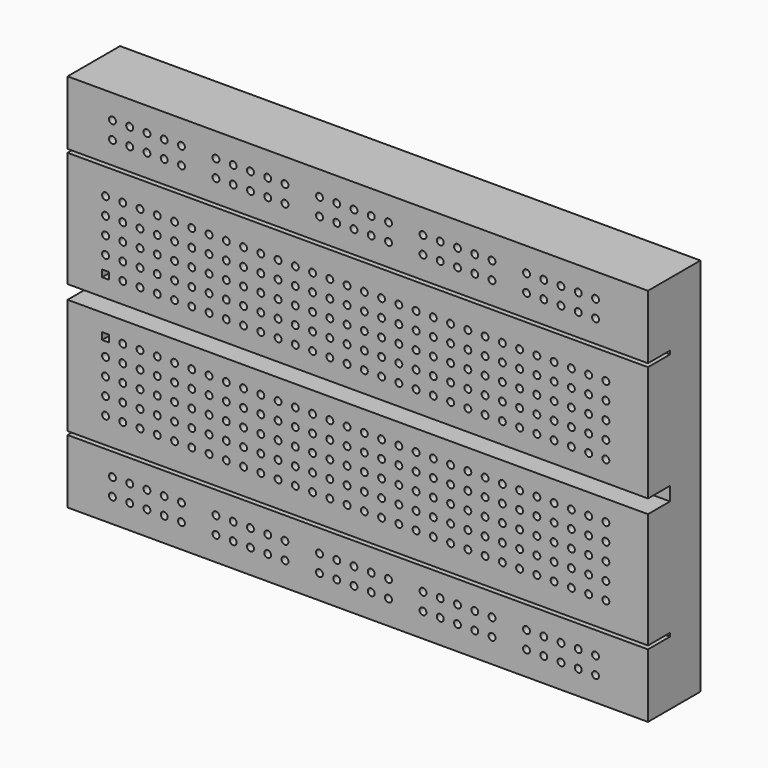
from build123d import *

# Parameters (mm, degrees)
F0_W     = 84.1
F0_H     = 55
F1_DEPTH = 9.5
F3_DEPTH = 5
F5_W     = 84.1
F5_H     = 2
F5_R     = 0.5
F5_H_2   = 0.5
F6_DEPTH = 4


with BuildPart() as f1:
    # F0 (on Front) → F1 (new body)
    with BuildSketch(Plane.XZ):
        Rectangle(F0_W, F0_H)
    extrude(amount=F1_DEPTH)

    # F2 (on face) → F3 (join)
    with BuildSketch(Plane(origin=(0, 0, 0), x_dir=(-1, 0, 0), z_dir=(0, 1, 0))):
        Polygon((44.05, 0), (42.05, 0), (42.05, -0.75), (44.05, -1.5), align=None)
        Polygon((44.05, 1.5), (42.05, 0.75), (42.05, 0), (44.05, 0), align=None)
        Polygon((1.5, -29.5), (0.75, -27.5), (-0.75, -27.5), (-1.5, -29.5), align=None)
    extrude(amount=-F3_DEPTH)

    # F5 (on face) → F6 (cut)
    with BuildSketch(Plane.XZ.offset(9.5)):
        Rectangle(F5_W, F5_H)
        with BuildLine():
            Line((-36.05, -4), (-36.05, -3.5))
            Line((-36.05, -3.5), (-36.55, -3.5))
            ThreePointArc((-36.55, -3.5), (-36.1964466094, -3.6464466094), (-36.05, -4))
        make_face()
        with BuildLine():
            ThreePointArc((-37.05, -4), (-36.9035533906, -3.6464466094), (-36.55, -3.5))
            Line((-36.55, -3.5), (-37.05, -3.5))
            Line((-37.05, -3.5), (-37.05, -4))
        make_face()
        with BuildLine():
            ThreePointArc((-36.05, -4), (-36.1964466094, -3.6464466094), (-36.55, -3.5))
            ThreePointArc((-36.55, -3.5), (-36.9035533906, -3.6464466094), (-37.05, -4))
            ThreePointArc((-37.05, -4), (-36.9035533906, -4.3535533906), (-36.55, -4.5))
            ThreePointArc((-36.55, -4.5), (-36.1964466094, -4.3535533906), (-36.05, -4))
        make_face()
        with BuildLine():
            Line((-36.05, -4.5), (-36.05, -4))
            ThreePointArc((-36.05, -4), (-36.1964466094, -4.3535533906), (-36.55, -4.5))
            Line((-36.55, -4.5), (-36.05, -4.5))
        make_face()
        with BuildLine():
            ThreePointArc((-36.55, -4.5), (-36.9035533906, -4.3535533906), (-37.05, -4))
            Line((-37.05, -4), (-37.05, -4.5))
            Line((-37.05, -4.5), (-36.55, -4.5))
        make_face()
        with Locations((-34.05, -4)):
            Circle(F5_R)
        with Locations((-31.55, -4)):
            Circle(F5_R)
        with Locations((-29.05, -4)):
            Circle(F5_R)
        with Locations((-26.55, -4)):
            Circle(F5_R)
        with Locations((-24.05, -4)):
            Circle(F5_R)
        with Locations((-21.55, -4)):
            Circle(F5_R)
        with Locations((-19.05, -4)):
            Circle(F5_R)
        with Locations((-16.55, -4)):
            Circle(F5_R)
        with Locations((-14.05, -4)):
            Circle(F5_R)
        with Locations((-11.55, -4)):
            Circle(F5_R)
        with Locations((-9.05, -4)):
            Circle(F5_R)
        with Locations((-6.55, -4)):
            Circle(F5_R)
        with Locations((-4.05, -4)):
            Circle(F5_R)
        with Locations((-1.55, -4)):
            Circle(F5_R)
        with Locations((0.95, -4)):
            Circle(F5_R)
        with Locations((3.45, -4)):
            Circle(F5_R)
        with Locations((5.95, -4)):
            Circle(F5_R)
        with Locations((8.45, -4)):
            Circle(F5_R)
        with Locations((10.95, -4)):
            Circle(F5_R)
        with Locations((13.45, -4)):
            Circle(F5_R)
        with Locations((15.95, -4)):
            Circle(F5_R)
        with Locations((18.45, -4)):
            Circle(F5_R)
        with Locations((20.95, -4)):
            Circle(F5_R)
        with Locations((23.45, -4)):
            Circle(F5_R)
        with Locations((25.95, -4)):
            Circle(F5_R)
        with Locations((28.45, -4)):
            Circle(F5_R)
        with Locations((30.95, -4)):
            Circle(F5_R)
        with Locations((33.45, -4)):
            Circle(F5_R)
        with Locations((35.95, -4)):
            Circle(F5_R)
        with Locations((25.95, -6.5)):
            Circle(F5_R)
        with Locations((28.45, -6.5)):
            Circle(F5_R)
        with Locations((-16.55, -6.5)):
            Circle(F5_R)
        with Locations((5.95, -6.5)):
            Circle(F5_R)
        with Locations((-31.55, -6.5)):
            Circle(F5_R)
        with Locations((20.95, -6.5)):
            Circle(F5_R)
        with Locations((-9.05, -6.5)):
            Circle(F5_R)
        with Locations((10.95, -6.5)):
            Circle(F5_R)
        with Locations((0.95, -6.5)):
            Circle(F5_R)
        with Locations((8.45, -6.5)):
            Circle(F5_R)
        with Locations((-14.05, -6.5)):
            Circle(F5_R)
        with Locations((-4.05, -6.5)):
            Circle(F5_R)
        with Locations((-11.55, -6.5)):
            Circle(F5_R)
        with Locations((15.95, -6.5)):
            Circle(F5_R)
        with Locations((3.45, -6.5)):
            Circle(F5_R)
        with Locations((13.45, -6.5)):
            Circle(F5_R)
        with Locations((-6.55, -6.5)):
            Circle(F5_R)
        with Locations((-29.05, -6.5)):
            Circle(F5_R)
        with Locations((18.45, -6.5)):
            Circle(F5_R)
        with Locations((23.45, -6.5)):
            Circle(F5_R)
        with Locations((30.95, -6.5)):
            Circle(F5_R)
        with Locations((33.45, -6.5)):
            Circle(F5_R)
        with Locations((-21.55, -6.5)):
            Circle(F5_R)
        with Locations((-26.55, -6.5)):
            Circle(F5_R)
        with Locations((-24.05, -6.5)):
            Circle(F5_R)
        with Locations((-19.05, -6.5)):
            Circle(F5_R)
        with Locations((35.95, -6.5)):
            Circle(F5_R)
        with Locations((-1.55, -6.5)):
            Circle(F5_R)
        with Locations((-34.05, -6.5)):
            Circle(F5_R)
        with Locations((-36.55, -6.5)):
            Circle(F5_R)
        with Locations((25.95, -9)):
            Circle(F5_R)
        with Locations((28.45, -9)):
            Circle(F5_R)
        with Locations((-16.55, -9)):
            Circle(F5_R)
        with Locations((5.95, -9)):
            Circle(F5_R)
        with Locations((-31.55, -9)):
            Circle(F5_R)
        with Locations((20.95, -9)):
            Circle(F5_R)
        with Locations((-9.05, -9)):
            Circle(F5_R)
        with Locations((10.95, -9)):
            Circle(F5_R)
        with Locations((0.95, -9)):
            Circle(F5_R)
        with Locations((8.45, -9)):
            Circle(F5_R)
        with Locations((-14.05, -9)):
            Circle(F5_R)
        with Locations((-4.05, -9)):
            Circle(F5_R)
        with Locations((-11.55, -9)):
            Circle(F5_R)
        with Locations((15.95, -9)):
            Circle(F5_R)
        with Locations((3.45, -9)):
            Circle(F5_R)
        with Locations((13.45, -9)):
            Circle(F5_R)
        with Locations((-6.55, -9)):
            Circle(F5_R)
        with Locations((-29.05, -9)):
            Circle(F5_R)
        with Locations((18.45, -9)):
            Circle(F5_R)
        with Locations((23.45, -9)):
            Circle(F5_R)
        with Locations((30.95, -9)):
            Circle(F5_R)
        with Locations((33.45, -9)):
            Circle(F5_R)
        with Locations((-21.55, -9)):
            Circle(F5_R)
        with Locations((-26.55, -9)):
            Circle(F5_R)
        with Locations((-24.05, -9)):
            Circle(F5_R)
        with Locations((-19.05, -9)):
            Circle(F5_R)
        with Locations((35.95, -9)):
            Circle(F5_R)
        with Locations((-1.55, -9)):
            Circle(F5_R)
        with Locations((-34.05, -9)):
            Circle(F5_R)
        with Locations((-36.55, -9)):
            Circle(F5_R)
        with Locations((25.95, -11.5)):
            Circle(F5_R)
        with Locations((28.45, -11.5)):
            Circle(F5_R)
        with Locations((-16.55, -11.5)):
            Circle(F5_R)
        with Locations((5.95, -11.5)):
            Circle(F5_R)
        with Locations((-31.55, -11.5)):
            Circle(F5_R)
        with Locations((20.95, -11.5)):
            Circle(F5_R)
        with Locations((-9.05, -11.5)):
            Circle(F5_R)
        with Locations((10.95, -11.5)):
            Circle(F5_R)
        with Locations((0.95, -11.5)):
            Circle(F5_R)
        with Locations((8.45, -11.5)):
            Circle(F5_R)
        with Locations((-14.05, -11.5)):
            Circle(F5_R)
        with Locations((-4.05, -11.5)):
            Circle(F5_R)
        with Locations((-11.55, -11.5)):
            Circle(F5_R)
        with Locations((15.95, -11.5)):
            Circle(F5_R)
        with Locations((3.45, -11.5)):
            Circle(F5_R)
        with Locations((13.45, -11.5)):
            Circle(F5_R)
        with Locations((-6.55, -11.5)):
            Circle(F5_R)
        with Locations((-29.05, -11.5)):
            Circle(F5_R)
        with Locations((18.45, -11.5)):
            Circle(F5_R)
        with Locations((23.45, -11.5)):
            Circle(F5_R)
        with Locations((30.95, -11.5)):
            Circle(F5_R)
        with Locations((33.45, -11.5)):
            Circle(F5_R)
        with Locations((-21.55, -11.5)):
            Circle(F5_R)
        with Locations((-26.55, -11.5)):
            Circle(F5_R)
        with Locations((-24.05, -11.5)):
            Circle(F5_R)
        with Locations((-19.05, -11.5)):
            Circle(F5_R)
        with Locations((35.95, -11.5)):
            Circle(F5_R)
        with Locations((-1.55, -11.5)):
            Circle(F5_R)
        with Locations((-34.05, -11.5)):
            Circle(F5_R)
        with Locations((-36.55, -11.5)):
            Circle(F5_R)
        with Locations((25.95, -14)):
            Circle(F5_R)
        with Locations((28.45, -14)):
            Circle(F5_R)
        with Locations((-16.55, -14)):
            Circle(F5_R)
        with Locations((5.95, -14)):
            Circle(F5_R)
        with Locations((-31.55, -14)):
            Circle(F5_R)
        with Locations((20.95, -14)):
            Circle(F5_R)
        with Locations((-9.05, -14)):
            Circle(F5_R)
        with Locations((10.95, -14)):
            Circle(F5_R)
        with Locations((0.95, -14)):
            Circle(F5_R)
        with Locations((8.45, -14)):
            Circle(F5_R)
        with Locations((-14.05, -14)):
            Circle(F5_R)
        with Locations((-4.05, -14)):
            Circle(F5_R)
        with Locations((-11.55, -14)):
            Circle(F5_R)
        with Locations((15.95, -14)):
            Circle(F5_R)
        with Locations((3.45, -14)):
            Circle(F5_R)
        with Locations((13.45, -14)):
            Circle(F5_R)
        with Locations((-6.55, -14)):
            Circle(F5_R)
        with Locations((-29.05, -14)):
            Circle(F5_R)
        with Locations((18.45, -14)):
            Circle(F5_R)
        with Locations((23.45, -14)):
            Circle(F5_R)
        with Locations((30.95, -14)):
            Circle(F5_R)
        with Locations((33.45, -14)):
            Circle(F5_R)
        with Locations((-21.55, -14)):
            Circle(F5_R)
        with Locations((-26.55, -14)):
            Circle(F5_R)
        with Locations((-24.05, -14)):
            Circle(F5_R)
        with Locations((-19.05, -14)):
            Circle(F5_R)
        with Locations((35.95, -14)):
            Circle(F5_R)
        with Locations((-1.55, -14)):
            Circle(F5_R)
        with Locations((-34.05, -14)):
            Circle(F5_R)
        with Locations((-36.55, -14)):
            Circle(F5_R)
        with Locations((0, -18)):
            Rectangle(F5_W, F5_H_2)
        with Locations((-35.55, -21.5)):
            Circle(F5_R)
        with Locations((-35.55, -24)):
            Circle(F5_R)
        with Locations((-33.05, -21.5)):
            Circle(F5_R)
        with Locations((-33.05, -24)):
            Circle(F5_R)
        with Locations((-30.55, -21.5)):
            Circle(F5_R)
        with Locations((-30.55, -24)):
            Circle(F5_R)
        with Locations((-28.05, -21.5)):
            Circle(F5_R)
        with Locations((-28.05, -24)):
            Circle(F5_R)
        with Locations((-25.55, -21.5)):
            Circle(F5_R)
        with Locations((-25.55, -24)):
            Circle(F5_R)
        with Locations((-18.05, -24)):
            Circle(F5_R)
        with Locations((-10.55, -24)):
            Circle(F5_R)
        with Locations((-13.05, -21.5)):
            Circle(F5_R)
        with Locations((-18.05, -21.5)):
            Circle(F5_R)
        with Locations((-15.55, -21.5)):
            Circle(F5_R)
        with Locations((-20.55, -24)):
            Circle(F5_R)
        with Locations((-13.05, -24)):
            Circle(F5_R)
        with Locations((-10.55, -21.5)):
            Circle(F5_R)
        with Locations((-15.55, -24)):
            Circle(F5_R)
        with Locations((-20.55, -21.5)):
            Circle(F5_R)
        with Locations((-3.05, -24)):
            Circle(F5_R)
        with Locations((4.45, -24)):
            Circle(F5_R)
        with Locations((1.95, -21.5)):
            Circle(F5_R)
        with Locations((-3.05, -21.5)):
            Circle(F5_R)
        with Locations((-0.55, -21.5)):
            Circle(F5_R)
        with Locations((-5.55, -24)):
            Circle(F5_R)
        with Locations((1.95, -24)):
            Circle(F5_R)
        with Locations((4.45, -21.5)):
            Circle(F5_R)
        with Locations((-0.55, -24)):
            Circle(F5_R)
        with Locations((-5.55, -21.5)):
            Circle(F5_R)
        with Locations((11.95, -24)):
            Circle(F5_R)
        with Locations((19.45, -24)):
            Circle(F5_R)
        with Locations((16.95, -21.5)):
            Circle(F5_R)
        with Locations((11.95, -21.5)):
            Circle(F5_R)
        with Locations((14.45, -21.5)):
            Circle(F5_R)
        with Locations((9.45, -24)):
            Circle(F5_R)
        with Locations((16.95, -24)):
            Circle(F5_R)
        with Locations((19.45, -21.5)):
            Circle(F5_R)
        with Locations((14.45, -24)):
            Circle(F5_R)
        with Locations((9.45, -21.5)):
            Circle(F5_R)
        with Locations((26.95, -24)):
            Circle(F5_R)
        with Locations((34.45, -24)):
            Circle(F5_R)
        with Locations((31.95, -21.5)):
            Circle(F5_R)
        with Locations((26.95, -21.5)):
            Circle(F5_R)
        with Locations((29.45, -21.5)):
            Circle(F5_R)
        with Locations((24.45, -24)):
            Circle(F5_R)
        with Locations((31.95, -24)):
            Circle(F5_R)
        with Locations((34.45, -21.5)):
            Circle(F5_R)
        with Locations((29.45, -24)):
            Circle(F5_R)
        with Locations((24.45, -21.5)):
            Circle(F5_R)
        with BuildLine():
            Line((-36.55, 3.5), (-36.05, 3.5))
            Line((-36.05, 3.5), (-36.05, 4))
            ThreePointArc((-36.05, 4), (-36.1964466094, 3.6464466094), (-36.55, 3.5))
        make_face()
        with BuildLine():
            Line((-37.05, 3.5), (-36.55, 3.5))
            ThreePointArc((-36.55, 3.5), (-36.9035533906, 3.6464466094), (-37.05, 4))
            Line((-37.05, 4), (-37.05, 3.5))
        make_face()
        with BuildLine():
            ThreePointArc((-37.05, 4), (-36.9035533906, 3.6464466094), (-36.55, 3.5))
            ThreePointArc((-36.55, 3.5), (-36.1964466094, 3.6464466094), (-36.05, 4))
            ThreePointArc((-36.05, 4), (-36.1964466094, 4.3535533906), (-36.55, 4.5))
            ThreePointArc((-36.55, 4.5), (-36.9035533906, 4.3535533906), (-37.05, 4))
        make_face()
        with BuildLine():
            ThreePointArc((-36.55, 4.5), (-36.1964466094, 4.3535533906), (-36.05, 4))
            Line((-36.05, 4), (-36.05, 4.5))
            Line((-36.05, 4.5), (-36.55, 4.5))
        make_face()
        with BuildLine():
            Line((-37.05, 4.5), (-37.05, 4))
            ThreePointArc((-37.05, 4), (-36.9035533906, 4.3535533906), (-36.55, 4.5))
            Line((-36.55, 4.5), (-37.05, 4.5))
        make_face()
        with Locations((-35.55, 21.5)):
            Circle(F5_R)
        with Locations((24.45, 21.5)):
            Circle(F5_R)
        with Locations((-20.55, 21.5)):
            Circle(F5_R)
        with Locations((-36.55, 6.5)):
            Circle(F5_R)
        with Locations((-5.55, 21.5)):
            Circle(F5_R)
        with Locations((9.45, 21.5)):
            Circle(F5_R)
        with Locations((-20.55, 24)):
            Circle(F5_R)
        with Locations((-35.55, 24)):
            Circle(F5_R)
        with Locations((-36.55, 11.5)):
            Circle(F5_R)
        with Locations((-3.05, 21.5)):
            Circle(F5_R)
        with Locations((-5.55, 24)):
            Circle(F5_R)
        with Locations((-36.55, 9)):
            Circle(F5_R)
        with Locations((26.95, 21.5)):
            Circle(F5_R)
        with Locations((-11.55, 4)):
            Circle(F5_R)
        with Locations((0, 18)):
            Rectangle(F5_W, F5_H_2)
        with Locations((11.95, 21.5)):
            Circle(F5_R)
        with Locations((-18.05, 21.5)):
            Circle(F5_R)
        with Locations((-34.05, 4)):
            Circle(F5_R)
        with Locations((-36.55, 14)):
            Circle(F5_R)
        with Locations((9.45, 24)):
            Circle(F5_R)
        with Locations((24.45, 24)):
            Circle(F5_R)
        with Locations((-33.05, 21.5)):
            Circle(F5_R)
        with Locations((-18.05, 24)):
            Circle(F5_R)
        with Locations((3.45, 4)):
            Circle(F5_R)
        with Locations((-26.55, 9)):
            Circle(F5_R)
        with Locations((20.95, 11.5)):
            Circle(F5_R)
        with Locations((-26.55, 6.5)):
            Circle(F5_R)
        with Locations((-29.05, 6.5)):
            Circle(F5_R)
        with Locations((25.95, 11.5)):
            Circle(F5_R)
        with Locations((30.95, 9)):
            Circle(F5_R)
        with Locations((-10.55, 24)):
            Circle(F5_R)
        with Locations((-21.55, 9)):
            Circle(F5_R)
        with Locations((35.95, 9)):
            Circle(F5_R)
        with Locations((-21.55, 14)):
            Circle(F5_R)
        with Locations((16.95, 21.5)):
            Circle(F5_R)
        with Locations((30.95, 4)):
            Circle(F5_R)
        with Locations((-11.55, 6.5)):
            Circle(F5_R)
        with Locations((-19.05, 6.5)):
            Circle(F5_R)
        with Locations((-9.05, 4)):
            Circle(F5_R)
        with Locations((25.95, 9)):
            Circle(F5_R)
        with Locations((-28.05, 24)):
            Circle(F5_R)
        with Locations((-31.55, 14)):
            Circle(F5_R)
        with Locations((-19.05, 14)):
            Circle(F5_R)
        with Locations((-4.05, 4)):
            Circle(F5_R)
        with Locations((-14.05, 11.5)):
            Circle(F5_R)
        with Locations((-24.05, 9)):
            Circle(F5_R)
        with Locations((29.45, 21.5)):
            Circle(F5_R)
        with Locations((-31.55, 6.5)):
            Circle(F5_R)
        with Locations((-33.05, 24)):
            Circle(F5_R)
        with Locations((25.95, 14)):
            Circle(F5_R)
        with Locations((-1.55, 14)):
            Circle(F5_R)
        with Locations((-24.05, 4)):
            Circle(F5_R)
        with Locations((-19.05, 4)):
            Circle(F5_R)
        with Locations((5.95, 14)):
            Circle(F5_R)
        with Locations((-14.05, 9)):
            Circle(F5_R)
        with Locations((-1.55, 11.5)):
            Circle(F5_R)
        with Locations((-16.55, 14)):
            Circle(F5_R)
        with Locations((-26.55, 4)):
            Circle(F5_R)
        with Locations((-29.05, 4)):
            Circle(F5_R)
        with Locations((33.45, 6.5)):
            Circle(F5_R)
        with Locations((3.45, 6.5)):
            Circle(F5_R)
        with Locations((-25.55, 24)):
            Circle(F5_R)
        with Locations((3.45, 14)):
            Circle(F5_R)
        with Locations((13.45, 6.5)):
            Circle(F5_R)
        with Locations((-24.05, 11.5)):
            Circle(F5_R)
        with Locations((-30.55, 24)):
            Circle(F5_R)
        with Locations((28.45, 6.5)):
            Circle(F5_R)
        with Locations((23.45, 9)):
            Circle(F5_R)
        with Locations((-26.55, 11.5)):
            Circle(F5_R)
        with Locations((5.95, 9)):
            Circle(F5_R)
        with Locations((10.95, 14)):
            Circle(F5_R)
        with Locations((29.45, 24)):
            Circle(F5_R)
        with Locations((15.95, 9)):
            Circle(F5_R)
        with Locations((13.45, 4)):
            Circle(F5_R)
        with Locations((-6.55, 11.5)):
            Circle(F5_R)
        with Locations((0.95, 14)):
            Circle(F5_R)
        with Locations((-31.55, 4)):
            Circle(F5_R)
        with Locations((-29.05, 9)):
            Circle(F5_R)
        with Locations((-13.05, 21.5)):
            Circle(F5_R)
        with Locations((35.95, 6.5)):
            Circle(F5_R)
        with Locations((30.95, 11.5)):
            Circle(F5_R)
        with Locations((-21.55, 4)):
            Circle(F5_R)
        with Locations((-24.05, 6.5)):
            Circle(F5_R)
        with Locations((8.45, 11.5)):
            Circle(F5_R)
        with Locations((-16.55, 4)):
            Circle(F5_R)
        with Locations((13.45, 9)):
            Circle(F5_R)
        with Locations((-4.05, 6.5)):
            Circle(F5_R)
        with Locations((15.95, 11.5)):
            Circle(F5_R)
        with Locations((-6.55, 4)):
            Circle(F5_R)
        with Locations((-6.55, 6.5)):
            Circle(F5_R)
        with Locations((-16.55, 9)):
            Circle(F5_R)
        with Locations((-4.05, 11.5)):
            Circle(F5_R)
        with Locations((18.45, 14)):
            Circle(F5_R)
        with Locations((5.95, 6.5)):
            Circle(F5_R)
        with Locations((19.45, 21.5)):
            Circle(F5_R)
        with Locations((0.95, 11.5)):
            Circle(F5_R)
        with Locations((-1.55, 4)):
            Circle(F5_R)
        with Locations((-4.05, 14)):
            Circle(F5_R)
        with Locations((31.95, 24)):
            Circle(F5_R)
        with Locations((-26.55, 14)):
            Circle(F5_R)
        with Locations((10.95, 11.5)):
            Circle(F5_R)
        with Locations((-1.55, 6.5)):
            Circle(F5_R)
        with Locations((15.95, 14)):
            Circle(F5_R)
        with Locations((-10.55, 21.5)):
            Circle(F5_R)
        with Locations((5.95, 11.5)):
            Circle(F5_R)
        with Locations((15.95, 6.5)):
            Circle(F5_R)
        with Locations((-0.55, 24)):
            Circle(F5_R)
        with Locations((33.45, 11.5)):
            Circle(F5_R)
        with Locations((28.45, 11.5)):
            Circle(F5_R)
        with Locations((-0.55, 21.5)):
            Circle(F5_R)
        with Locations((0.95, 4)):
            Circle(F5_R)
        with Locations((8.45, 4)):
            Circle(F5_R)
        with Locations((25.95, 6.5)):
            Circle(F5_R)
        with Locations((-11.55, 11.5)):
            Circle(F5_R)
        with Locations((-28.05, 21.5)):
            Circle(F5_R)
        with Locations((-9.05, 11.5)):
            Circle(F5_R)
        with Locations((13.45, 11.5)):
            Circle(F5_R)
        with Locations((20.95, 14)):
            Circle(F5_R)
        with Locations((8.45, 6.5)):
            Circle(F5_R)
        with Locations((-24.05, 14)):
            Circle(F5_R)
        with Locations((-6.55, 14)):
            Circle(F5_R)
        with Locations((-30.55, 21.5)):
            Circle(F5_R)
        with Locations((23.45, 4)):
            Circle(F5_R)
        with Locations((19.45, 24)):
            Circle(F5_R)
        with Locations((-11.55, 14)):
            Circle(F5_R)
        with Locations((18.45, 9)):
            Circle(F5_R)
        with Locations((-34.05, 11.5)):
            Circle(F5_R)
        with Locations((28.45, 14)):
            Circle(F5_R)
        with Locations((35.95, 14)):
            Circle(F5_R)
        with Locations((35.95, 4)):
            Circle(F5_R)
        with Locations((-4.05, 9)):
            Circle(F5_R)
        with Locations((33.45, 9)):
            Circle(F5_R)
        with Locations((20.95, 9)):
            Circle(F5_R)
        with Locations((33.45, 14)):
            Circle(F5_R)
        with Locations((34.45, 24)):
            Circle(F5_R)
        with Locations((35.95, 11.5)):
            Circle(F5_R)
        with Locations((14.45, 24)):
            Circle(F5_R)
        with Locations((-31.55, 9)):
            Circle(F5_R)
        with Locations((0.95, 9)):
            Circle(F5_R)
        with Locations((18.45, 11.5)):
            Circle(F5_R)
        with Locations((-13.05, 24)):
            Circle(F5_R)
        with Locations((4.45, 21.5)):
            Circle(F5_R)
        with Locations((28.45, 9)):
            Circle(F5_R)
        with Locations((8.45, 14)):
            Circle(F5_R)
        with Locations((1.95, 21.5)):
            Circle(F5_R)
        with Locations((-21.55, 6.5)):
            Circle(F5_R)
        with Locations((3.45, 11.5)):
            Circle(F5_R)
        with Locations((-9.05, 9)):
            Circle(F5_R)
        with Locations((-19.05, 9)):
            Circle(F5_R)
        with Locations((-16.55, 11.5)):
            Circle(F5_R)
        with Locations((5.95, 4)):
            Circle(F5_R)
        with Locations((-34.05, 14)):
            Circle(F5_R)
        with Locations((18.45, 4)):
            Circle(F5_R)
        with Locations((-9.05, 14)):
            Circle(F5_R)
        with Locations((-19.05, 11.5)):
            Circle(F5_R)
        with Locations((-1.55, 9)):
            Circle(F5_R)
        with Locations((-34.05, 9)):
            Circle(F5_R)
        with Locations((23.45, 6.5)):
            Circle(F5_R)
        with Locations((30.95, 14)):
            Circle(F5_R)
        with Locations((-6.55, 9)):
            Circle(F5_R)
        with Locations((13.45, 14)):
            Circle(F5_R)
        with Locations((-34.05, 6.5)):
            Circle(F5_R)
        with Locations((16.95, 24)):
            Circle(F5_R)
        with Locations((-25.55, 21.5)):
            Circle(F5_R)
        with Locations((-14.05, 6.5)):
            Circle(F5_R)
        with Locations((-14.05, 4)):
            Circle(F5_R)
        with Locations((3.45, 9)):
            Circle(F5_R)
        with Locations((31.95, 21.5)):
            Circle(F5_R)
        with Locations((10.95, 6.5)):
            Circle(F5_R)
        with Locations((18.45, 6.5)):
            Circle(F5_R)
        with Locations((-29.05, 11.5)):
            Circle(F5_R)
        with Locations((28.45, 4)):
            Circle(F5_R)
        with Locations((14.45, 21.5)):
            Circle(F5_R)
        with Locations((-15.55, 21.5)):
            Circle(F5_R)
        with Locations((10.95, 4)):
            Circle(F5_R)
        with Locations((33.45, 4)):
            Circle(F5_R)
        with Locations((-9.05, 6.5)):
            Circle(F5_R)
        with Locations((10.95, 9)):
            Circle(F5_R)
        with Locations((15.95, 4)):
            Circle(F5_R)
        with Locations((-14.05, 14)):
            Circle(F5_R)
        with Locations((23.45, 14)):
            Circle(F5_R)
        with Locations((-29.05, 14)):
            Circle(F5_R)
        with Locations((20.95, 6.5)):
            Circle(F5_R)
        with Locations((-21.55, 11.5)):
            Circle(F5_R)
        with Locations((-11.55, 9)):
            Circle(F5_R)
        with Locations((1.95, 24)):
            Circle(F5_R)
        with Locations((23.45, 11.5)):
            Circle(F5_R)
        with Locations((-3.05, 24)):
            Circle(F5_R)
        with Locations((8.45, 9)):
            Circle(F5_R)
        with Locations((25.95, 4)):
            Circle(F5_R)
        with Locations((34.45, 21.5)):
            Circle(F5_R)
        with Locations((-16.55, 6.5)):
            Circle(F5_R)
        with Locations((20.95, 4)):
            Circle(F5_R)
        with Locations((26.95, 24)):
            Circle(F5_R)
        with Locations((0.95, 6.5)):
            Circle(F5_R)
        with Locations((11.95, 24)):
            Circle(F5_R)
        with Locations((4.45, 24)):
            Circle(F5_R)
        with Locations((30.95, 6.5)):
            Circle(F5_R)
        with Locations((-31.55, 11.5)):
            Circle(F5_R)
        with Locations((-15.55, 24)):
            Circle(F5_R)
    extrude(amount=-F6_DEPTH, mode=Mode.SUBTRACT)


solid = f1.part
